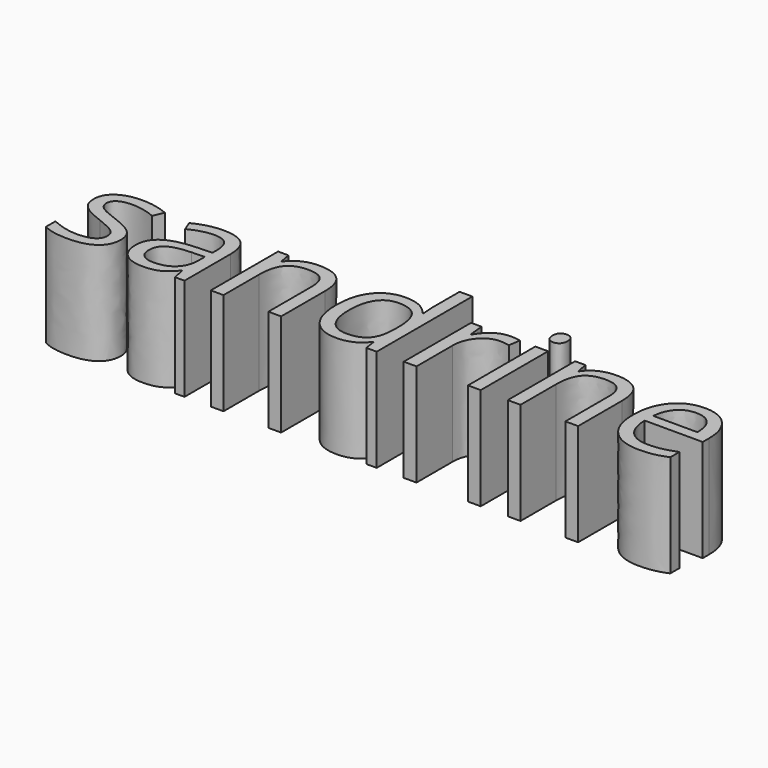
from build123d import *

# Parameters (mm, degrees)
F0_TEXT_SIZE = 76.8975872133
F1_DEPTH     = 50


# Not quite as in the source:
# - Text() gives the source's letters only with a copy of the font that has no kerning and outlines rounded to 1/6400 em; it was checked with that copy


with BuildPart() as f1:
    # F0 (on Top) → F1 (new body)
    with BuildSketch(Plane.XY):
        with Locations((-315.9169157184, -55.3662627935)):
            Text('sandrine', F0_TEXT_SIZE, font='Open Sans', text_align=(TextAlign.LEFT, TextAlign.BOTTOM))
    extrude(amount=F1_DEPTH)


solid = f1.part
